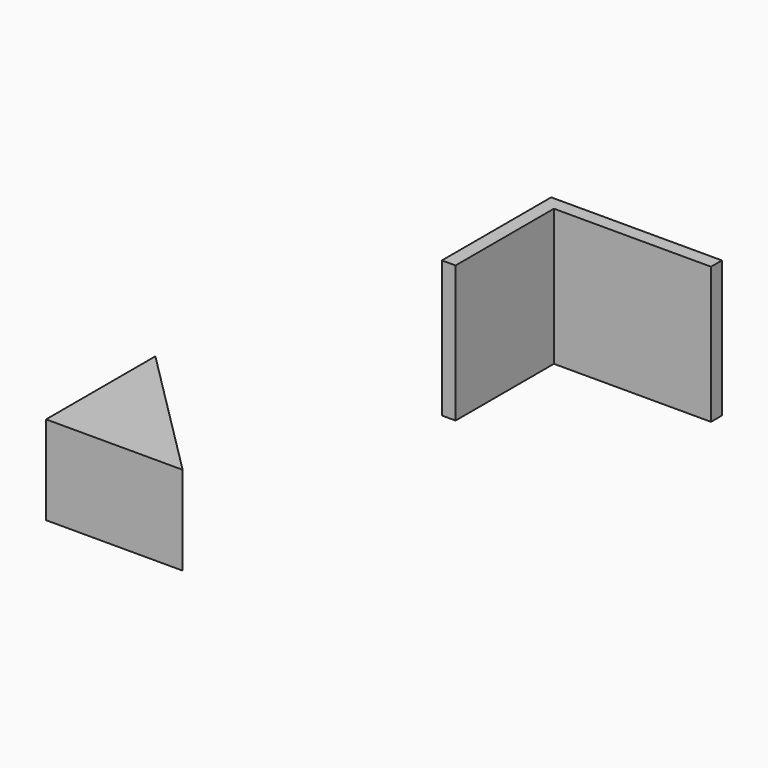
from build123d import *

# Parameters (mm, degrees)
F0_W     = 31.75
F0_H     = 25.4
F1_DEPTH = 25.4
F2_T     = -2.54
F4_DEPTH = 19.05
F6_DEPTH = 2.54
F6_TAPER = -5


with BuildPart() as f1:
    # F0 (on Front) → F1 (new body)
    with BuildSketch(Plane.XZ):
        with Locations((15.875, 19.3175956197)):
            Rectangle(F0_W, F0_H)
    extrude(amount=F1_DEPTH)

    # F2
    f2_openings = [f1.faces().sort_by_distance(p)[0] for p in [
        (15.875, -25.4, 19.317596),
        (31.75, -12.7, 19.317596),
        (15.875, -12.7, 6.617596),
        (15.875, -12.7, 32.017596),
    ]]
    offset(amount=F2_T, openings=f2_openings)


with BuildPart() as f4:
    # F3 (on Top) → F4 (new body)
    with BuildSketch(Plane.XY):
        Polygon((-55.1244552851, -23.1033010297), (-55.1244552851, -48.5033010297), (-29.7244552851, -48.5033010297), align=None)
    extrude(amount=F4_DEPTH)


with BuildPart() as f4_1:
    # F5: moved
    add(f4.part.moved(Location((0, 0, -19.05))))

    # F4_face (on face) → F6 (cut)
    with BuildSketch(Plane(origin=(-46.6577886184, -40.036634363, 0), x_dir=(1, 0, 0), z_dir=(0, 0, 1))):
        Polygon((16.9333333333, -8.4666666667), (-8.4666666667, 16.9333333333), (-8.4666666667, -8.4666666667), align=None)
    extrude(amount=-F6_DEPTH, taper=F6_TAPER, mode=Mode.SUBTRACT)


solid = Compound([f1.part, f4_1.part])
